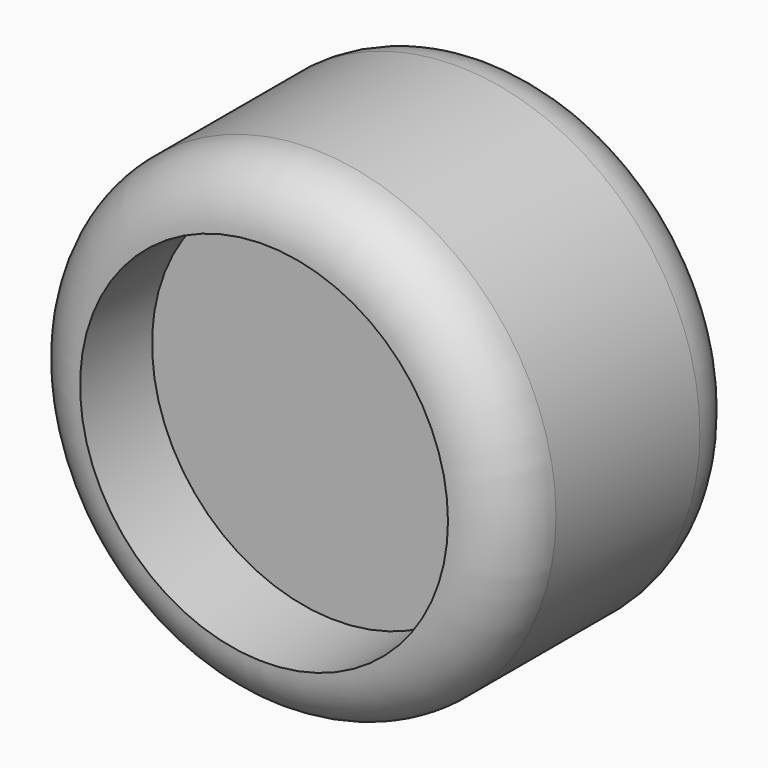
from build123d import *

# Parameters (mm, degrees)
F4_R     = 20.6580157973
F5_DEPTH = 12.7
F6_DEPTH = 12.7
F7_R     = 5.08
F8_DEPTH = 7.62
F9_DEPTH = 7.62


# Not quite as in the source:
# - a feature of the source that left no trace in its solid (it failed there, or was rolled back) is left out


with BuildPart() as f5:
    # F4 (on Front) → F5 (new body)
    with BuildSketch(Plane.XZ):
        with Locations((0, -189.9833083153)):
            Circle(F4_R)
    extrude(amount=F5_DEPTH)

    # F6 (add): a face of the model
    f6_faces = [f5.faces().sort_by_distance(p)[0] for p in [
        (0, 0, -189.9833083153),
    ]]
    extrude(f6_faces, amount=F6_DEPTH)

    # F7
    f7_edges = [f5.edges().sort_by_distance(p)[0] for p in [
        (-20.658016, -12.7, -189.983308),
        (-20.658016, 12.7, -189.983308),
    ]]
    fillet(f7_edges, radius=F7_R)

    # F8 (cut): a face of the model
    f8_faces = [f5.faces().sort_by_distance(p)[0] for p in [
        (0, -12.7, -189.9833083153),
    ]]
    extrude(f8_faces, amount=-F8_DEPTH, mode=Mode.SUBTRACT)

    # F9 (cut): a face of the model
    f9_faces = [f5.faces().sort_by_distance(p)[0] for p in [
        (0, 12.7, -189.9833083153),
    ]]
    extrude(f9_faces, amount=-F9_DEPTH, mode=Mode.SUBTRACT)


solid = f5.part
